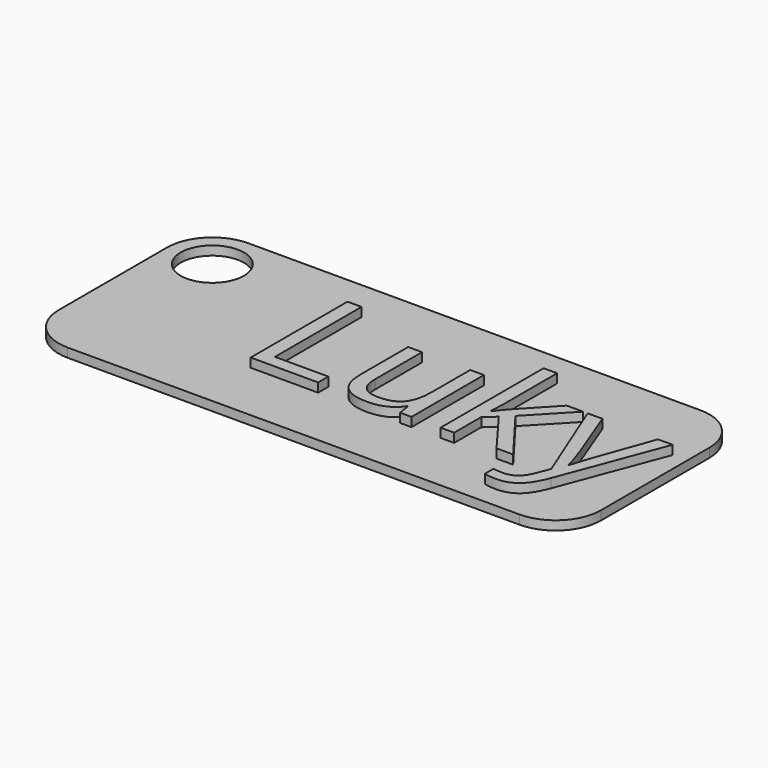
from build123d import *

# Parameters (mm, degrees)
F0_W         = 60
F0_H         = 25
F1_DEPTH     = 1
F2_TEXT_SIZE = 18.7500004864
F3_DEPTH     = 1
F4_R         = 5
F6_D         = 7
F6_DEPTH     = 50
F6_TIP       = 2.1030121666


# Not quite as in the source:
# - Text() gives the source's letters only with a copy of the font that has no kerning and outlines rounded to 1/6400 em; it was checked with that copy


with BuildPart() as f1:
    # F0 (on Top) → F1 (new body)
    with BuildSketch(Plane.XY):
        Rectangle(F0_W, F0_H)
    extrude(amount=F1_DEPTH)

    # F2 (on face) → F3 (join)
    with BuildSketch(Plane.XY.offset(1)):
        with Locations((-12.1304367203, -5.5760871619)):
            Text('Luky', F2_TEXT_SIZE, font='Open Sans', text_align=(TextAlign.LEFT, TextAlign.BOTTOM))
    extrude(amount=F3_DEPTH)

    # F4
    f4_edges = [f1.edges().sort_by_distance(p)[0] for p in [
        (-30, 12.5, 0.5),
        (-30, -12.5, 0.5),
        (30, -12.5, 0.5),
        (30, 12.5, 0.5),
    ]]
    fillet(f4_edges, radius=F4_R)

    # F6
    with Locations(Plane.XY.offset(1)):
        with Locations((-25, 7.5)):
            Hole(F6_D / 2, depth=F6_DEPTH)
            with Locations((0, 0, -(F6_DEPTH + F6_TIP / 2))):  # 118° drill point
                Cone(0, F6_D / 2, F6_TIP, mode=Mode.SUBTRACT)


solid = f1.part
